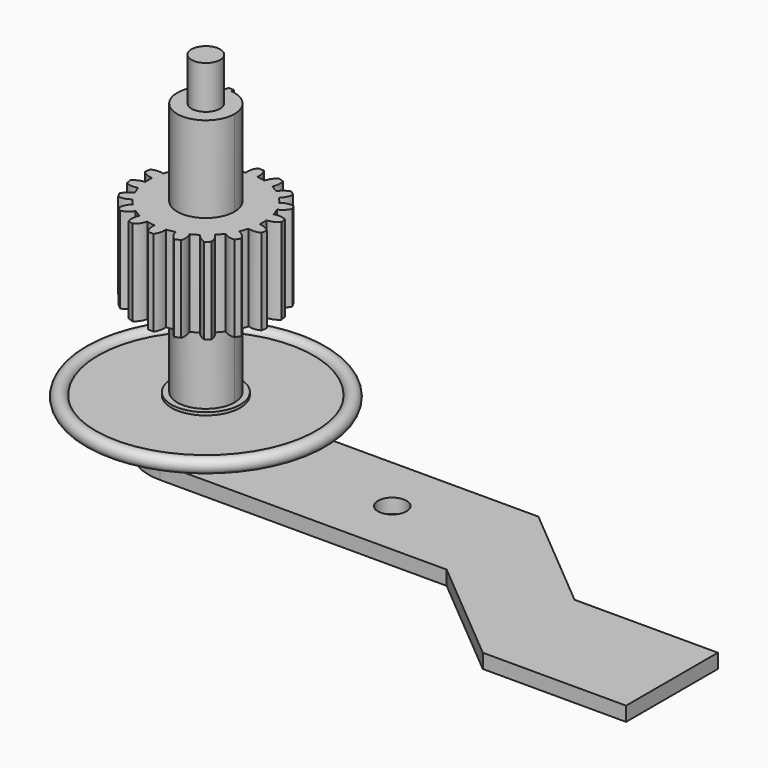
from build123d import *

# Parameters (mm, degrees)
F1_DEPTH  = 15
F0_R      = 5
F2_DEPTH  = 60
F3_COUNT  = 18
F4_DEPTH  = 45
F9_DEPTH  = 3.9
F10_R     = 5
F11_DEPTH = 2.5


with BuildPart() as f1:
    # F0 (on Top) → F1 (new body, symmetric)
    with BuildSketch(Plane.XY):
        with BuildLine():
            ThreePointArc((-1, 24), (-1.8724139119, 22.0407014664), (-2, 19.8997487421))
            ThreePointArc((-2, 19.8997487421), (0, -20), (2, 19.8997487421))
            ThreePointArc((2, 19.8997487421), (1.8724139119, 22.0407014664), (1, 24))
            Line((1, 24), (-1, 24))
        make_face()
        with BuildLine():
            ThreePointArc((1, 9.9498743711), (7.4161984871, 6.7082039325), (10, 0))
            ThreePointArc((10, 0), (-6.7082039325, -7.4161984871), (-1, 9.9498743711))
            Line((-1, 9.9498743711), (-1, 11))
            Line((-1, 11), (1, 11))
            Line((1, 11), (1, 9.9498743711))
        make_face(mode=Mode.SUBTRACT)
    extrude(amount=F1_DEPTH, both=True)

    # F3: F1 ×18 about axis
    f3_axis = Axis((0, 0, 0), (0, 0, 1))


with BuildPart() as f2:
    # F0 (on Top) → F2 (new body, symmetric)
    with BuildSketch(Plane.XY):
        Circle(F0_R)
    extrude(amount=F2_DEPTH, both=True)


with BuildPart() as f1_1:
    add(f1.part)
    for i in range(1, F3_COUNT):
        add(f1.part.rotate(f3_axis, i * 360 / F3_COUNT))

    # F0 (on Top) → F4 (join, symmetric)
    with BuildSketch(Plane.XY):
        with BuildLine():
            Line((1, 9), (1, 9.9498743711))
            ThreePointArc((1, 9.9498743711), (0, 10), (-1, 9.9498743711))
            Line((-1, 9.9498743711), (-1, 9))
            Line((-1, 9), (1, 9))
        make_face()
        with BuildLine():
            ThreePointArc((-1, 9.9498743711), (-6.7082039325, -7.4161984871), (10, 0))
            ThreePointArc((10, 0), (7.4161984871, 6.7082039325), (1, 9.9498743711))
            Line((1, 9.9498743711), (1, 9))
            Line((1, 9), (-1, 9))
            Line((-1, 9), (-1, 9.9498743711))
        make_face()
        Circle(F0_R, mode=Mode.SUBTRACT)
        with BuildLine():
            ThreePointArc((-1, 9.9498743711), (0, 10), (1, 9.9498743711))
            Line((1, 9.9498743711), (1, 11))
            Line((1, 11), (-1, 11))
            Line((-1, 11), (-1, 9.9498743711))
        make_face()
        with BuildLine():
            ThreePointArc((-1, 9.9498743711), (-6.7082039325, -7.4161984871), (10, 0))
            ThreePointArc((10, 0), (7.4161984871, 6.7082039325), (1, 9.9498743711))
            Line((1, 9.9498743711), (1, 9))
            Line((1, 9), (-1, 9))
            Line((-1, 9), (-1, 9.9498743711))
        make_face()
        Circle(F0_R, mode=Mode.SUBTRACT)
    extrude(amount=F4_DEPTH, both=True)


with BuildPart() as f7:
    # F6 (on Front) → F7 (revolve)
    with BuildSketch(Plane.XZ):
        with BuildLine():
            ThreePointArc((-37.5203414348, -45.4127976298), (-37.4946192857, -45.2071107576), (-37.486025542, -45))
            ThreePointArc((-37.486025542, -45), (-37.4946192857, -44.7928892424), (-37.5203414348, -44.5872023702))
            ThreePointArc((-37.5203414348, -44.5872023702), (-42.486025542, -45), (-37.5203414348, -45.4127976298))
        make_face()
        with BuildLine():
            ThreePointArc((-37.5203414348, -44.5872023702), (-37.4946192857, -44.7928892424), (-37.486025542, -45))
            ThreePointArc((-37.486025542, -45), (-37.4946192857, -45.2071107576), (-37.5203414348, -45.4127976298))
            Line((-37.5203414348, -45.4127976298), (-12, -45.4127976298))
            Line((-12, -45.4127976298), (-12, -46.4127976298))
            Line((-12, -46.4127976298), (-10, -46.4127976298))
            Line((-10, -46.4127976298), (-10, -45))
            Line((-10, -45), (-10, -43.5872023702))
            Line((-10, -43.5872023702), (-12, -43.5872023702))
            Line((-12, -43.5872023702), (-12, -44.5872023702))
            Line((-12, -44.5872023702), (-37.5203414348, -44.5872023702))
        make_face()
    revolve(axis=Axis((0, 0, -45), (0, 0, -1)))

    # F8 (on face) → F9 (cut, symmetric)
    with BuildSketch(Plane(origin=(0, 0, -45.4127976298), x_dir=(1, 0, 0), z_dir=(0, 0, -1))):
        Polygon((1, -11), (1, -9.9498743711), (1, -9), (-1, -9), (-1, -9.9498743711), (-1, -11), align=None)
    extrude(amount=F9_DEPTH, both=True, mode=Mode.SUBTRACT)


with BuildPart() as f11:
    # F10 (on face) → F11 (new body, symmetric)
    with BuildSketch(Plane(origin=(0, 0, -60), x_dir=(1, 0, 0), z_dir=(0, 0, -1))):
        with BuildLine():
            ThreePointArc((0, -20), (14.1421356237, -14.1421356237), (20, 0))
            ThreePointArc((20, 0), (14.1421356237, 14.1421356237), (0, 20))
            ThreePointArc((0, 20), (-20, 0), (0, -20))
        make_face()
        Circle(F10_R, mode=Mode.SUBTRACT)
        with BuildLine():
            ThreePointArc((0, 20), (14.1421356237, 14.1421356237), (20, 0))
            ThreePointArc((20, 0), (14.1421356237, -14.1421356237), (0, -20))
            Line((0, -20), (100, -20))
            Line((100, -20), (138.3022221559, 12.1393804843))
            Line((138.3022221559, 12.1393804843), (188.3022221559, 12.1393804843))
            Line((188.3022221559, 12.1393804843), (188.3022221559, 52.1393804843))
            Line((188.3022221559, 52.1393804843), (138.3022221559, 52.1393804843))
            Line((138.3022221559, 52.1393804843), (100, 20))
            Line((100, 20), (0, 20))
        make_face()
        with Locations((65, 0)):
            Circle(F10_R, mode=Mode.SUBTRACT)
    extrude(amount=F11_DEPTH, both=True)


solid = Compound([f2.part, f1_1.part, f7.part, f11.part])
